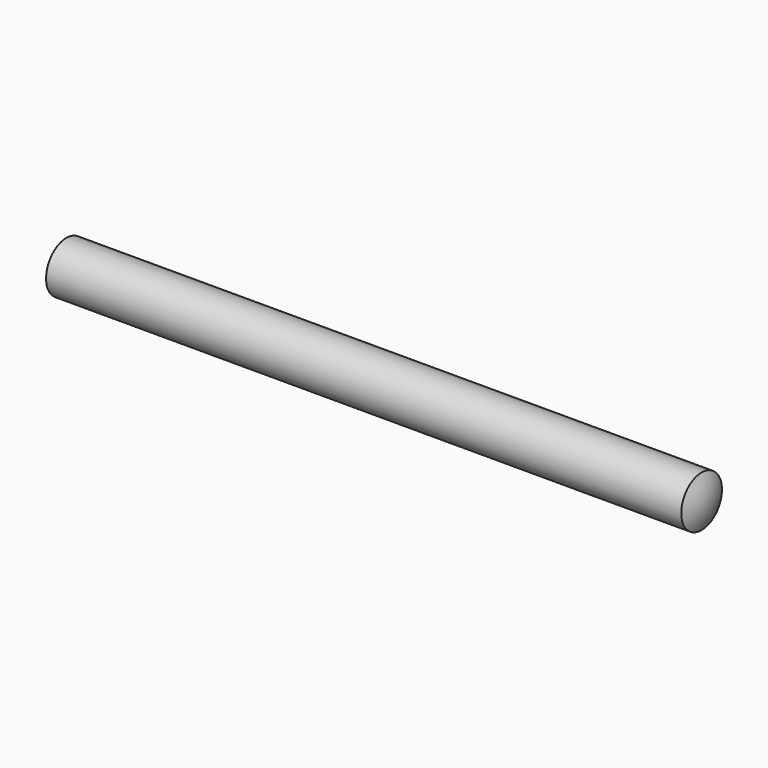
from build123d import *

# Parameters (mm, degrees)
F0_R     = 4
F1_DEPTH = 50


# Not quite as in the source:
# - a pattern or mirror of a feature is missing from the dataset's text; its kind, count and spacing are read off the source's solid


with BuildPart() as f1:
    # F0 (on Right) → F1 (new body, symmetric)
    with BuildSketch(Plane.YZ):
        Circle(F0_R)
    extrude(amount=F1_DEPTH, both=True)

    # F2 (on Front) → F3 (revolve)
    with BuildSketch(Plane.XZ):
        with BuildLine():
            ThreePointArc((51.0717967697, 0), (50.79920338, 2.0705523608), (50, 4))
            Line((50, 4), (50, 0))
            Line((50, 0), (51.0717967697, 0))
        make_face()
    f3 = revolve(axis=Axis((0, 0, 0), (1, 0, 0)))

    # F3_copies: F3 across plane
    add(f3.mirror(Plane(origin=(0, 0, 0), x_dir=(0, 0, -1), z_dir=(-1, 0, 0))))


solid = f1.part
